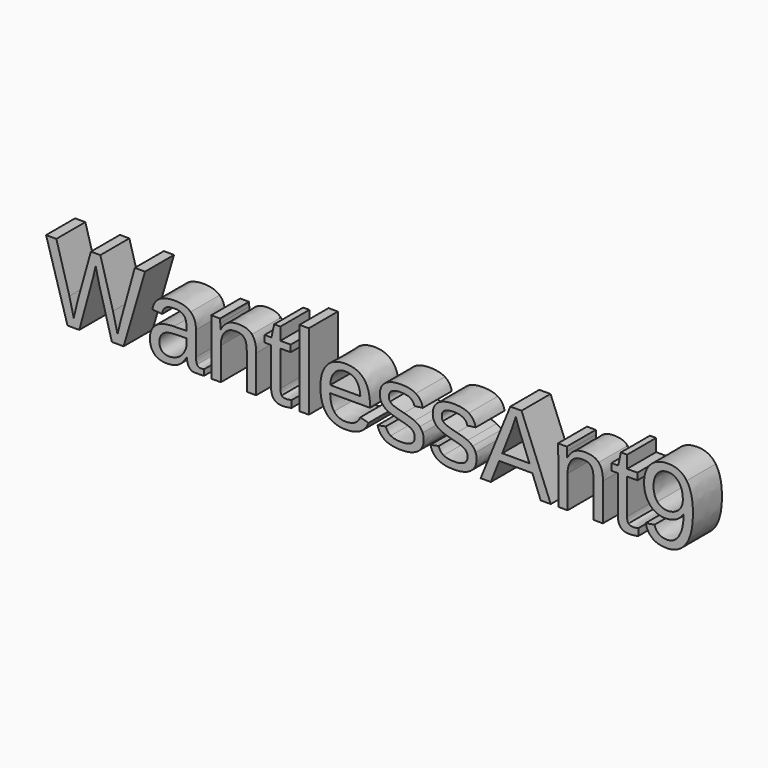
from build123d import *

# Parameters (mm, degrees)
F0_W     = 2.5657552083
F0_H     = 21
F1_DEPTH = 10


with BuildPart() as f1:
    # F0 (on Front) → F1 (new body)
    with BuildSketch(Plane.XZ):
        with BuildLine():
            Line((79.0343266088, 10), (83.371302383, 10))
            add(Edge.make_bspline(
                [(86.66796875, 12.4905598958), (85.3878334896, 10.605916318), (83.371302383, 10)],
                knots=[0, 0, 0, 0.6784981919, 0.6784981919, 0.6784981919], degree=2))
            add(Edge.make_bspline(
                [(88.5546875, 20.4407552083), (88.5546875, 15.2682291667), (86.66796875, 12.4905598958)],
                knots=[0, 0, 0, 1, 1, 1], degree=2))
            add(Edge.make_bspline(
                [(86.83203125, 27.8873697917), (88.5546875, 25.408203125), (88.5546875, 20.4407552083)],
                knots=[0, 0, 0, 1, 1, 1], degree=2))
            add(Edge.make_bspline(
                [(81.7643229167, 30.3665364583), (85.109375, 30.3665364583), (86.83203125, 27.8873697917)],
                knots=[0, 0, 0, 1, 1, 1], degree=2))
            add(Edge.make_bspline(
                [(76.8492838542, 28.5641276042), (78.615234375, 30.3665364583), (81.7643229167, 30.3665364583)],
                knots=[0, 0, 0, 1, 1, 1], degree=2))
            add(Edge.make_bspline(
                [(75.0833333333, 23.6171875), (75.0833333333, 26.76171875), (76.8492838542, 28.5641276042)],
                knots=[0, 0, 0, 1, 1, 1], degree=2))
            add(Edge.make_bspline(
                [(76.7080078125, 18.7021484375), (75.0833333333, 20.5546875), (75.0833333333, 23.6171875)],
                knots=[0, 0, 0, 1, 1, 1], degree=2))
            add(Edge.make_bspline(
                [(81.03515625, 16.849609375), (78.3326822917, 16.849609375), (76.7080078125, 18.7021484375)],
                knots=[0, 0, 0, 1, 1, 1], degree=2))
            add(Edge.make_bspline(
                [(84.0703125, 17.6266276042), (82.689453125, 16.849609375), (81.03515625, 16.849609375)],
                knots=[0, 0, 0, 1, 1, 1], degree=2))
            add(Edge.make_bspline(
                [(86.0208333333, 19.6842447917), (85.451171875, 18.4036458333), (84.0703125, 17.6266276042)],
                knots=[0, 0, 0, 1, 1, 1], degree=2))
            add(Edge.make_bspline(
                [(84.75390625, 13.8326822917), (85.9661458333, 15.8834635417), (86.0208333333, 19.6842447917)],
                knots=[0, 0, 0, 1, 1, 1], degree=2))
            add(Edge.make_bspline(
                [(81.3359375, 11.7819010417), (83.5416666667, 11.7819010417), (84.75390625, 13.8326822917)],
                knots=[0, 0, 0, 1, 1, 1], degree=2))
            add(Edge.make_bspline(
                [(77.9453125, 14.2884114583), (78.7154947917, 11.7819010417), (81.3359375, 11.7819010417)],
                knots=[0, 0, 0, 1, 1, 1], degree=2))
            Line((77.9453125, 14.2884114583), (75.498046875, 13.9010416667))
            add(Edge.make_bspline(
                [(77.5260416667, 10.7041015625), (76.1087239583, 11.6953125), (75.498046875, 13.9010416667)],
                knots=[0, 0, 0, 1, 1, 1], degree=2))
            add(Edge.make_bspline(
                [(79.0343266088, 10), (78.1805643403, 10.2463566059), (77.5260416667, 10.7041015625)],
                knots=[0.5381962211, 0.5381962211, 0.5381962211, 1, 1, 1], degree=2))
        make_face()
        with BuildLine():
            add(Edge.make_bspline(
                [(85.765625, 22.9153645833), (85.765625, 25.33984375), (84.6536458333, 26.8141276042)],
                knots=[0, 0, 0, 1, 1, 1], degree=2))
            add(Edge.make_bspline(
                [(85.2164713542, 20.8098958333), (85.765625, 21.7350260417), (85.765625, 22.9153645833)],
                knots=[0, 0, 0, 1, 1, 1], degree=2))
            add(Edge.make_bspline(
                [(83.7125651042, 19.37890625), (84.6673177083, 19.884765625), (85.2164713542, 20.8098958333)],
                knots=[0, 0, 0, 1, 1, 1], degree=2))
            add(Edge.make_bspline(
                [(81.650390625, 18.873046875), (82.7578125, 18.873046875), (83.7125651042, 19.37890625)],
                knots=[0, 0, 0, 1, 1, 1], degree=2))
            add(Edge.make_bspline(
                [(78.7587890625, 20.1468098958), (79.8274739583, 18.873046875), (81.650390625, 18.873046875)],
                knots=[0, 0, 0, 1, 1, 1], degree=2))
            add(Edge.make_bspline(
                [(77.6901041667, 23.6171875), (77.6901041667, 21.4205729167), (78.7587890625, 20.1468098958)],
                knots=[0, 0, 0, 1, 1, 1], degree=2))
            add(Edge.make_bspline(
                [(78.7587890625, 27.0260416667), (77.6901041667, 25.763671875), (77.6901041667, 23.6171875)],
                knots=[0, 0, 0, 1, 1, 1], degree=2))
            add(Edge.make_bspline(
                [(81.677734375, 28.2884114583), (79.8274739583, 28.2884114583), (78.7587890625, 27.0260416667)],
                knots=[0, 0, 0, 1, 1, 1], degree=2))
            add(Edge.make_bspline(
                [(84.6536458333, 26.8141276042), (83.5416666667, 28.2884114583), (81.677734375, 28.2884114583)],
                knots=[0, 0, 0, 1, 1, 1], degree=2))
        make_face(mode=Mode.SUBTRACT)
        with BuildLine():
            add(Edge.make_bspline(
                [(83.371302383, 10), (82.4157826709, 9.712890625), (81.294921875, 9.712890625)],
                knots=[0.6784981919, 0.6784981919, 0.6784981919, 1, 1, 1], degree=2))
            Line((83.371302383, 10), (79.0343266088, 10))
            add(Edge.make_bspline(
                [(81.294921875, 9.712890625), (80.0293198238, 9.712890625), (79.0343266088, 10)],
                knots=[0, 0, 0, 0.5381962211, 0.5381962211, 0.5381962211], degree=2))
        make_face()
        with BuildLine():
            add(Edge.make_bspline(
                [(73.0351407022, 10), (71.9925052469, 9.7721354167), (70.9134114583, 9.7721354167)],
                knots=[0.1835034191, 0.1835034191, 0.1835034191, 1, 1, 1], degree=2))
            Line((73.0351407022, 10), (69.5423555663, 10))
            add(Edge.make_bspline(
                [(70.9134114583, 9.7721354167), (70.1274862579, 9.7721354167), (69.5423555663, 10)],
                knots=[0, 0, 0, 0.2554880652, 0.2554880652, 0.2554880652], degree=2))
        make_face()
        with BuildLine():
            Line((69.5423555663, 10), (73.0351407022, 10))
            add(Edge.make_bspline(
                [(73.501953125, 10.1139322917), (73.2694676735, 10.0512113965), (73.0351407022, 10)],
                knots=[0, 0, 0, 0.1835034191, 0.1835034191, 0.1835034191], degree=2))
            Line((73.501953125, 10.1139322917), (73.501953125, 12.009765625))
            add(Edge.make_bspline(
                [(72.0208333333, 11.8092447917), (72.5358072917, 11.8092447917), (73.501953125, 12.009765625)],
                knots=[0, 0, 0, 1, 1, 1], degree=2))
            add(Edge.make_bspline(
                [(70.7607421875, 12.2581380208), (71.123046875, 11.8092447917), (72.0208333333, 11.8092447917)],
                knots=[0, 0, 0, 1, 1, 1], degree=2))
            add(Edge.make_bspline(
                [(70.3984375, 13.8190104167), (70.3984375, 12.70703125), (70.7607421875, 12.2581380208)],
                knots=[0, 0, 0, 1, 1, 1], degree=2))
            Line((70.3984375, 13.8190104167), (70.3984375, 23.5442708333))
            Line((70.3984375, 23.5442708333), (73.2467447917, 23.5442708333))
            Line((73.2467447917, 23.5442708333), (73.2467447917, 25.408203125))
            Line((73.2467447917, 25.408203125), (70.3984375, 25.408203125))
            Line((70.3984375, 25.408203125), (70.3984375, 28.8580729167))
            Line((70.3984375, 28.8580729167), (68.689453125, 28.8580729167))
            Line((68.689453125, 28.8580729167), (67.9329427083, 25.408203125))
            Line((67.9329427083, 25.408203125), (66.0553385417, 25.408203125))
            Line((66.0553385417, 25.408203125), (66.0553385417, 23.5442708333))
            Line((66.0553385417, 23.5442708333), (67.8372395833, 23.5442708333))
            Line((67.8372395833, 23.5442708333), (67.8372395833, 13.2630208333))
            add(Edge.make_bspline(
                [(69.5423555663, 10), (67.8372395833, 10.6640149774), (67.8372395833, 13.2630208333)],
                knots=[0.2554880652, 0.2554880652, 0.2554880652, 1, 1, 1], degree=2))
        make_face()
        with BuildLine():
            Line((61.142578125, 10), (63.7220052083, 10))
            Line((63.7220052083, 10), (63.7220052083, 20.267578125))
            add(Edge.make_bspline(
                [(62.5462239583, 24.4352213542), (63.7220052083, 23.1751302083), (63.7220052083, 20.267578125)],
                knots=[0, 0, 0, 1, 1, 1], degree=2))
            add(Edge.make_bspline(
                [(58.8365885417, 25.6953125), (61.3704427083, 25.6953125), (62.5462239583, 24.4352213542)],
                knots=[0, 0, 0, 1, 1, 1], degree=2))
            add(Edge.make_bspline(
                [(55.9518229167, 25.0322265625), (57.1139322917, 25.6953125), (58.8365885417, 25.6953125)],
                knots=[0, 0, 0, 1, 1, 1], degree=2))
            add(Edge.make_bspline(
                [(53.91015625, 22.7740885417), (54.7897135417, 24.369140625), (55.9518229167, 25.0322265625)],
                knots=[0, 0, 0, 1, 1, 1], degree=2))
            Line((53.91015625, 22.7740885417), (53.8645833333, 22.7740885417))
            add(Edge.make_bspline(
                [(53.8167317708, 24.3053385417), (53.8372395833, 23.8997395833), (53.8645833333, 22.7740885417)],
                knots=[0, 0, 0, 1, 1, 1], degree=2))
            add(Edge.make_bspline(
                [(53.7802734375, 25.025390625), (53.7962239583, 24.7109375), (53.8167317708, 24.3053385417)],
                knots=[0, 0, 0, 1, 1, 1], degree=2))
            add(Edge.make_bspline(
                [(53.7506510417, 25.408203125), (53.7643229167, 25.33984375), (53.7802734375, 25.025390625)],
                knots=[0, 0, 0, 1, 1, 1], degree=2))
            Line((53.7506510417, 25.408203125), (51.3307291667, 25.408203125))
            add(Edge.make_bspline(
                [(51.4173177083, 22.1178385417), (51.4173177083, 24.8111979167), (51.3307291667, 25.408203125)],
                knots=[0, 0, 0, 1, 1, 1], degree=2))
            Line((51.4173177083, 22.1178385417), (51.4173177083, 10))
            Line((51.4173177083, 10), (53.978515625, 10))
            Line((53.978515625, 10), (53.978515625, 18.927734375))
            add(Edge.make_bspline(
                [(55.0472005208, 22.4459635417), (53.978515625, 21.1790364583), (53.978515625, 18.927734375)],
                knots=[0, 0, 0, 1, 1, 1], degree=2))
            add(Edge.make_bspline(
                [(57.9661458333, 23.712890625), (56.1158854167, 23.712890625), (55.0472005208, 22.4459635417)],
                knots=[0, 0, 0, 1, 1, 1], degree=2))
            add(Edge.make_bspline(
                [(59.8893229167, 23.34375), (59.2330729167, 23.712890625), (57.9661458333, 23.712890625)],
                knots=[0, 0, 0, 1, 1, 1], degree=2))
            add(Edge.make_bspline(
                [(60.8440755208, 22.1337890625), (60.5455729167, 22.974609375), (59.8893229167, 23.34375)],
                knots=[0, 0, 0, 1, 1, 1], degree=2))
            add(Edge.make_bspline(
                [(61.142578125, 19.7708333333), (61.142578125, 21.29296875), (60.8440755208, 22.1337890625)],
                knots=[0, 0, 0, 1, 1, 1], degree=2))
            Line((61.142578125, 19.7708333333), (61.142578125, 10))
        make_face()
        Polygon((38.1829427083, 30.0657552083), (29.998046875, 10), (32.814453125, 10), (35.125, 15.8697916667), (44.2669270833, 15.8697916667), (46.5592447917, 10), (49.3346354167, 10), (41.27734375, 30.0657552083), align=None)
        with BuildLine():
            Line((39.568359375, 27.6184895833), (39.6959635417, 28.0149739583))
            Line((39.6959635417, 28.0149739583), (40.0787760417, 26.8346354167))
            add(Edge.make_bspline(
                [(40.8763020833, 24.6106770833), (40.4798177083, 25.5950520833), (40.0787760417, 26.8346354167)],
                knots=[0, 0, 0, 1, 1, 1], degree=2))
            Line((40.8763020833, 24.6106770833), (43.4557291667, 17.9889322917))
            Line((43.4557291667, 17.9889322917), (35.9498697917, 17.9889322917))
            Line((35.9498697917, 17.9889322917), (38.5110677083, 24.5833333333))
            add(Edge.make_bspline(
                [(39.568359375, 27.6184895833), (39.2083333333, 26.43359375), (38.5110677083, 24.5833333333)],
                knots=[0, 0, 0, 1, 1, 1], degree=2))
        make_face(mode=Mode.SUBTRACT)
        with BuildLine():
            add(Edge.make_bspline(
                [(19.8664633143, 10), (18.8987870961, 10.2345761258), (18.1969401042, 10.6608072917)],
                knots=[0.5503495393, 0.5503495393, 0.5503495393, 1, 1, 1], degree=2))
            Line((19.8664633143, 10), (25.2328343309, 10))
            add(Edge.make_bspline(
                [(27.2408854167, 10.8955078125), (26.4063199616, 10.2955916475), (25.2328343309, 10)],
                knots=[0, 0, 0, 0.5072784088, 0.5072784088, 0.5072784088], degree=2))
            add(Edge.make_bspline(
                [(28.8860677083, 14.2565104167), (28.8860677083, 12.078125), (27.2408854167, 10.8955078125)],
                knots=[0, 0, 0, 1, 1, 1], degree=2))
            add(Edge.make_bspline(
                [(28.6012369792, 15.8310546875), (28.8860677083, 15.140625), (28.8860677083, 14.2565104167)],
                knots=[0, 0, 0, 1, 1, 1], degree=2))
            add(Edge.make_bspline(
                [(27.796875, 17.0501302083), (28.31640625, 16.521484375), (28.6012369792, 15.8310546875)],
                knots=[0, 0, 0, 1, 1, 1], degree=2))
            add(Edge.make_bspline(
                [(26.3795572917, 18.01171875), (27.27734375, 17.5787760417), (27.796875, 17.0501302083)],
                knots=[0, 0, 0, 1, 1, 1], degree=2))
            add(Edge.make_bspline(
                [(23.4446614583, 18.9596354167), (25.4817708333, 18.4446614583), (26.3795572917, 18.01171875)],
                knots=[0, 0, 0, 1, 1, 1], degree=2))
            add(Edge.make_bspline(
                [(20.6236979167, 19.7845052083), (21.2936197917, 19.4837239583), (23.4446614583, 18.9596354167)],
                knots=[0, 0, 0, 1, 1, 1], degree=2))
            add(Edge.make_bspline(
                [(19.6119791667, 20.5113932292), (19.9537760417, 20.0852864583), (20.6236979167, 19.7845052083)],
                knots=[0, 0, 0, 1, 1, 1], degree=2))
            add(Edge.make_bspline(
                [(19.2701822917, 21.59375), (19.2701822917, 20.9375), (19.6119791667, 20.5113932292)],
                knots=[0, 0, 0, 1, 1, 1], degree=2))
            add(Edge.make_bspline(
                [(20.0973307292, 23.1865234375), (19.2701822917, 22.66015625), (19.2701822917, 21.59375)],
                knots=[0, 0, 0, 1, 1, 1], degree=2))
            add(Edge.make_bspline(
                [(22.6608072917, 23.712890625), (20.9244791667, 23.712890625), (20.0973307292, 23.1865234375)],
                knots=[0, 0, 0, 1, 1, 1], degree=2))
            add(Edge.make_bspline(
                [(25.1604817708, 23.166015625), (24.228515625, 23.712890625), (22.6608072917, 23.712890625)],
                knots=[0, 0, 0, 1, 1, 1], degree=2))
            add(Edge.make_bspline(
                [(26.306640625, 21.59375), (26.0924479167, 22.619140625), (25.1604817708, 23.166015625)],
                knots=[0, 0, 0, 1, 1, 1], degree=2))
            Line((26.306640625, 21.59375), (28.6126302083, 21.8763020833))
            add(Edge.make_bspline(
                [(26.7145182292, 24.7542317708), (28.2161458333, 23.8587239583), (28.6126302083, 21.8763020833)],
                knots=[0, 0, 0, 1, 1, 1], degree=2))
            add(Edge.make_bspline(
                [(22.6608072917, 25.6497395833), (25.212890625, 25.6497395833), (26.7145182292, 24.7542317708)],
                knots=[0, 0, 0, 1, 1, 1], degree=2))
            add(Edge.make_bspline(
                [(18.2835286458, 24.546875), (19.78515625, 25.6497395833), (22.6608072917, 25.6497395833)],
                knots=[0, 0, 0, 1, 1, 1], degree=2))
            add(Edge.make_bspline(
                [(16.7819010417, 21.3385416667), (16.7819010417, 23.4440104167), (18.2835286458, 24.546875)],
                knots=[0, 0, 0, 1, 1, 1], degree=2))
            add(Edge.make_bspline(
                [(17.3082682292, 19.4153645833), (16.7819010417, 20.19921875), (16.7819010417, 21.3385416667)],
                knots=[0, 0, 0, 1, 1, 1], degree=2))
            add(Edge.make_bspline(
                [(18.7666015625, 18.0823567708), (17.8346354167, 18.6315104167), (17.3082682292, 19.4153645833)],
                knots=[0, 0, 0, 1, 1, 1], degree=2))
            add(Edge.make_bspline(
                [(21.9088541667, 16.9635416667), (19.6985677083, 17.533203125), (18.7666015625, 18.0823567708)],
                knots=[0, 0, 0, 1, 1, 1], degree=2))
            Line((21.9088541667, 16.9635416667), (23.7454427083, 16.48046875))
            add(Edge.make_bspline(
                [(25.7666015625, 15.5416666667), (25.1399739583, 16.111328125), (23.7454427083, 16.48046875)],
                knots=[0, 0, 0, 1, 1, 1], degree=2))
            add(Edge.make_bspline(
                [(26.3932291667, 14.060546875), (26.3932291667, 14.9720052083), (25.7666015625, 15.5416666667)],
                knots=[0, 0, 0, 1, 1, 1], degree=2))
            add(Edge.make_bspline(
                [(25.4886067708, 12.2649739583), (26.3932291667, 12.8619791667), (26.3932291667, 14.060546875)],
                knots=[0, 0, 0, 1, 1, 1], degree=2))
            add(Edge.make_bspline(
                [(22.6334635417, 11.66796875), (24.583984375, 11.66796875), (25.4886067708, 12.2649739583)],
                knots=[0, 0, 0, 1, 1, 1], degree=2))
            add(Edge.make_bspline(
                [(19.78515625, 12.2444661458), (20.810546875, 11.66796875), (22.6334635417, 11.66796875)],
                knots=[0, 0, 0, 1, 1, 1], degree=2))
            add(Edge.make_bspline(
                [(18.431640625, 14.060546875), (18.759765625, 12.8209635417), (19.78515625, 12.2444661458)],
                knots=[0, 0, 0, 1, 1, 1], degree=2))
            Line((18.431640625, 14.060546875), (16.1666666667, 13.6184895833))
            add(Edge.make_bspline(
                [(18.1969401042, 10.6608072917), (16.6360677083, 11.6087239583), (16.1666666667, 13.6184895833)],
                knots=[0, 0, 0, 1, 1, 1], degree=2))
        make_face()
        with BuildLine():
            add(Edge.make_bspline(
                [(5.283129981, 10), (4.3154537627, 10.2345761258), (3.6136067708, 10.6608072917)],
                knots=[0.5503495393, 0.5503495393, 0.5503495393, 1, 1, 1], degree=2))
            Line((5.283129981, 10), (10.6495009976, 10))
            add(Edge.make_bspline(
                [(12.6575520833, 10.8955078125), (11.8229866283, 10.2955916475), (10.6495009976, 10)],
                knots=[0, 0, 0, 0.5072784088, 0.5072784088, 0.5072784088], degree=2))
            add(Edge.make_bspline(
                [(14.302734375, 14.2565104167), (14.302734375, 12.078125), (12.6575520833, 10.8955078125)],
                knots=[0, 0, 0, 1, 1, 1], degree=2))
            add(Edge.make_bspline(
                [(14.0179036458, 15.8310546875), (14.302734375, 15.140625), (14.302734375, 14.2565104167)],
                knots=[0, 0, 0, 1, 1, 1], degree=2))
            add(Edge.make_bspline(
                [(13.2135416667, 17.0501302083), (13.7330729167, 16.521484375), (14.0179036458, 15.8310546875)],
                knots=[0, 0, 0, 1, 1, 1], degree=2))
            add(Edge.make_bspline(
                [(11.7962239583, 18.01171875), (12.6940104167, 17.5787760417), (13.2135416667, 17.0501302083)],
                knots=[0, 0, 0, 1, 1, 1], degree=2))
            add(Edge.make_bspline(
                [(8.861328125, 18.9596354167), (10.8984375, 18.4446614583), (11.7962239583, 18.01171875)],
                knots=[0, 0, 0, 1, 1, 1], degree=2))
            add(Edge.make_bspline(
                [(6.0403645833, 19.7845052083), (6.7102864583, 19.4837239583), (8.861328125, 18.9596354167)],
                knots=[0, 0, 0, 1, 1, 1], degree=2))
            add(Edge.make_bspline(
                [(5.0286458333, 20.5113932292), (5.3704427083, 20.0852864583), (6.0403645833, 19.7845052083)],
                knots=[0, 0, 0, 1, 1, 1], degree=2))
            add(Edge.make_bspline(
                [(4.6868489583, 21.59375), (4.6868489583, 20.9375), (5.0286458333, 20.5113932292)],
                knots=[0, 0, 0, 1, 1, 1], degree=2))
            add(Edge.make_bspline(
                [(5.5139973958, 23.1865234375), (4.6868489583, 22.66015625), (4.6868489583, 21.59375)],
                knots=[0, 0, 0, 1, 1, 1], degree=2))
            add(Edge.make_bspline(
                [(8.0774739583, 23.712890625), (6.3411458333, 23.712890625), (5.5139973958, 23.1865234375)],
                knots=[0, 0, 0, 1, 1, 1], degree=2))
            add(Edge.make_bspline(
                [(10.5771484375, 23.166015625), (9.6451822917, 23.712890625), (8.0774739583, 23.712890625)],
                knots=[0, 0, 0, 1, 1, 1], degree=2))
            add(Edge.make_bspline(
                [(11.7233072917, 21.59375), (11.5091145833, 22.619140625), (10.5771484375, 23.166015625)],
                knots=[0, 0, 0, 1, 1, 1], degree=2))
            Line((11.7233072917, 21.59375), (14.029296875, 21.8763020833))
            add(Edge.make_bspline(
                [(12.1311848958, 24.7542317708), (13.6328125, 23.8587239583), (14.029296875, 21.8763020833)],
                knots=[0, 0, 0, 1, 1, 1], degree=2))
            add(Edge.make_bspline(
                [(8.0774739583, 25.6497395833), (10.6295572917, 25.6497395833), (12.1311848958, 24.7542317708)],
                knots=[0, 0, 0, 1, 1, 1], degree=2))
            add(Edge.make_bspline(
                [(3.7001953125, 24.546875), (5.2018229167, 25.6497395833), (8.0774739583, 25.6497395833)],
                knots=[0, 0, 0, 1, 1, 1], degree=2))
            add(Edge.make_bspline(
                [(2.1985677083, 21.3385416667), (2.1985677083, 23.4440104167), (3.7001953125, 24.546875)],
                knots=[0, 0, 0, 1, 1, 1], degree=2))
            add(Edge.make_bspline(
                [(2.7249348958, 19.4153645833), (2.1985677083, 20.19921875), (2.1985677083, 21.3385416667)],
                knots=[0, 0, 0, 1, 1, 1], degree=2))
            add(Edge.make_bspline(
                [(4.1832682292, 18.0823567708), (3.2513020833, 18.6315104167), (2.7249348958, 19.4153645833)],
                knots=[0, 0, 0, 1, 1, 1], degree=2))
            add(Edge.make_bspline(
                [(7.3255208333, 16.9635416667), (5.115234375, 17.533203125), (4.1832682292, 18.0823567708)],
                knots=[0, 0, 0, 1, 1, 1], degree=2))
            Line((7.3255208333, 16.9635416667), (9.162109375, 16.48046875))
            add(Edge.make_bspline(
                [(11.1832682292, 15.5416666667), (10.556640625, 16.111328125), (9.162109375, 16.48046875)],
                knots=[0, 0, 0, 1, 1, 1], degree=2))
            add(Edge.make_bspline(
                [(11.8098958333, 14.060546875), (11.8098958333, 14.9720052083), (11.1832682292, 15.5416666667)],
                knots=[0, 0, 0, 1, 1, 1], degree=2))
            add(Edge.make_bspline(
                [(10.9052734375, 12.2649739583), (11.8098958333, 12.8619791667), (11.8098958333, 14.060546875)],
                knots=[0, 0, 0, 1, 1, 1], degree=2))
            add(Edge.make_bspline(
                [(8.0501302083, 11.66796875), (10.0006510417, 11.66796875), (10.9052734375, 12.2649739583)],
                knots=[0, 0, 0, 1, 1, 1], degree=2))
            add(Edge.make_bspline(
                [(5.2018229167, 12.2444661458), (6.2272135417, 11.66796875), (8.0501302083, 11.66796875)],
                knots=[0, 0, 0, 1, 1, 1], degree=2))
            add(Edge.make_bspline(
                [(3.8483072917, 14.060546875), (4.1764322917, 12.8209635417), (5.2018229167, 12.2444661458)],
                knots=[0, 0, 0, 1, 1, 1], degree=2))
            Line((3.8483072917, 14.060546875), (1.5833333333, 13.6184895833))
            add(Edge.make_bspline(
                [(3.6136067708, 10.6608072917), (2.052734375, 11.6087239583), (1.5833333333, 13.6184895833)],
                knots=[0, 0, 0, 1, 1, 1], degree=2))
        make_face()
        with BuildLine():
            Line((25.2328343309, 10), (19.8664633143, 10))
            add(Edge.make_bspline(
                [(22.6334635417, 9.712890625), (21.0508503158, 9.712890625), (19.8664633143, 10)],
                knots=[0, 0, 0, 0.5503495393, 0.5503495393, 0.5503495393], degree=2))
            add(Edge.make_bspline(
                [(25.2328343309, 10), (24.0930229428, 9.712890625), (22.6334635417, 9.712890625)],
                knots=[0.5072784088, 0.5072784088, 0.5072784088, 1, 1, 1], degree=2))
        make_face()
        with BuildLine():
            Line((10.6495009976, 10), (5.283129981, 10))
            add(Edge.make_bspline(
                [(8.0501302083, 9.712890625), (6.4675169824, 9.712890625), (5.283129981, 10)],
                knots=[0, 0, 0, 0.5503495393, 0.5503495393, 0.5503495393], degree=2))
            add(Edge.make_bspline(
                [(10.6495009976, 10), (9.5096896095, 9.712890625), (8.0501302083, 9.712890625)],
                knots=[0.5072784088, 0.5072784088, 0.5072784088, 1, 1, 1], degree=2))
        make_face()
        with BuildLine():
            Line((-4.7456217987, 10), (-9.5531948379, 10))
            add(Edge.make_bspline(
                [(-7.216796875, 9.712890625), (-8.499968067, 9.712890625), (-9.5531948379, 10)],
                knots=[0, 0, 0, 0.3754192288, 0.3754192288, 0.3754192288], degree=2))
            add(Edge.make_bspline(
                [(-4.7456217987, 10), (-5.8428520101, 9.712890625), (-7.216796875, 9.712890625)],
                knots=[0.7195509219, 0.7195509219, 0.7195509219, 1, 1, 1], degree=2))
        make_face()
        with BuildLine():
            add(Edge.make_bspline(
                [(-9.5531948379, 10), (-11.3054364347, 10.4776606554), (-12.4212239583, 11.75)],
                knots=[0.3754192288, 0.3754192288, 0.3754192288, 1, 1, 1], degree=2))
            Line((-9.5531948379, 10), (-4.7456217987, 10))
            add(Edge.make_bspline(
                [(-0.9368489583, 13.36328125), (-1.9304475947, 10.7366393104), (-4.7456217987, 10)],
                knots=[0, 0, 0, 0.7195509219, 0.7195509219, 0.7195509219], degree=2))
            Line((-0.9368489583, 13.36328125), (-3.18359375, 14.0013020833))
            add(Edge.make_bspline(
                [(-4.5439453125, 12.3059895833), (-3.5390625, 12.9759114583), (-3.18359375, 14.0013020833)],
                knots=[0, 0, 0, 1, 1, 1], degree=2))
            add(Edge.make_bspline(
                [(-7.216796875, 11.6360677083), (-5.548828125, 11.6360677083), (-4.5439453125, 12.3059895833)],
                knots=[0, 0, 0, 1, 1, 1], degree=2))
            add(Edge.make_bspline(
                [(-10.4182942708, 13.076171875), (-9.322265625, 11.6360677083), (-7.216796875, 11.6360677083)],
                knots=[0, 0, 0, 1, 1, 1], degree=2))
            add(Edge.make_bspline(
                [(-11.5143229167, 17.1640625), (-11.5143229167, 14.5162760417), (-10.4182942708, 13.076171875)],
                knots=[0, 0, 0, 1, 1, 1], degree=2))
            Line((-11.5143229167, 17.1640625), (-0.5221354167, 17.1640625))
            Line((-0.5221354167, 17.1640625), (-0.5221354167, 17.505859375))
            add(Edge.make_bspline(
                [(-7.3170572917, 25.6953125), (-0.5221354167, 25.6953125), (-0.5221354167, 17.505859375)],
                knots=[0, 0, 0, 1, 1, 1], degree=2))
            add(Edge.make_bspline(
                [(-12.4212239583, 23.658203125), (-10.634765625, 25.6953125), (-7.3170572917, 25.6953125)],
                knots=[0, 0, 0, 1, 1, 1], degree=2))
            add(Edge.make_bspline(
                [(-14.2076822917, 17.806640625), (-14.2076822917, 21.62109375), (-12.4212239583, 23.658203125)],
                knots=[0, 0, 0, 1, 1, 1], degree=2))
            add(Edge.make_bspline(
                [(-12.4212239583, 11.75), (-14.2076822917, 13.787109375), (-14.2076822917, 17.806640625)],
                knots=[0, 0, 0, 1, 1, 1], degree=2))
        make_face()
        with BuildLine():
            add(Edge.make_bspline(
                [(-3.169921875, 19.1282552083), (-3.3841145833, 21.56640625), (-4.4095052083, 22.6829427083)],
                knots=[0, 0, 0, 1, 1, 1], degree=2))
            Line((-3.169921875, 19.1282552083), (-11.4869791667, 19.1282552083))
            add(Edge.make_bspline(
                [(-10.3111979167, 22.5530598958), (-11.400390625, 21.306640625), (-11.4869791667, 19.1282552083)],
                knots=[0, 0, 0, 1, 1, 1], degree=2))
            add(Edge.make_bspline(
                [(-7.3580729167, 23.7994791667), (-9.2220052083, 23.7994791667), (-10.3111979167, 22.5530598958)],
                knots=[0, 0, 0, 1, 1, 1], degree=2))
            add(Edge.make_bspline(
                [(-4.4095052083, 22.6829427083), (-5.4348958333, 23.7994791667), (-7.3580729167, 23.7994791667)],
                knots=[0, 0, 0, 1, 1, 1], degree=2))
        make_face(mode=Mode.SUBTRACT)
        with Locations((-18.6806640625, 20.5)):
            Rectangle(F0_W, F0_H)
        with BuildLine():
            Line((-26.101524642, 10), (-22.6087395061, 10))
            add(Edge.make_bspline(
                [(-22.1419270833, 10.1139322917), (-22.3744125348, 10.0512113965), (-22.6087395061, 10)],
                knots=[0, 0, 0, 0.1835034191, 0.1835034191, 0.1835034191], degree=2))
            Line((-22.1419270833, 10.1139322917), (-22.1419270833, 12.009765625))
            add(Edge.make_bspline(
                [(-23.623046875, 11.8092447917), (-23.1080729167, 11.8092447917), (-22.1419270833, 12.009765625)],
                knots=[0, 0, 0, 1, 1, 1], degree=2))
            add(Edge.make_bspline(
                [(-24.8831380208, 12.2581380208), (-24.5208333333, 11.8092447917), (-23.623046875, 11.8092447917)],
                knots=[0, 0, 0, 1, 1, 1], degree=2))
            add(Edge.make_bspline(
                [(-25.2454427083, 13.8190104167), (-25.2454427083, 12.70703125), (-24.8831380208, 12.2581380208)],
                knots=[0, 0, 0, 1, 1, 1], degree=2))
            Line((-25.2454427083, 13.8190104167), (-25.2454427083, 23.5442708333))
            Line((-25.2454427083, 23.5442708333), (-22.3971354167, 23.5442708333))
            Line((-22.3971354167, 23.5442708333), (-22.3971354167, 25.408203125))
            Line((-22.3971354167, 25.408203125), (-25.2454427083, 25.408203125))
            Line((-25.2454427083, 25.408203125), (-25.2454427083, 28.8580729167))
            Line((-25.2454427083, 28.8580729167), (-26.9544270833, 28.8580729167))
            Line((-26.9544270833, 28.8580729167), (-27.7109375, 25.408203125))
            Line((-27.7109375, 25.408203125), (-29.5885416667, 25.408203125))
            Line((-29.5885416667, 25.408203125), (-29.5885416667, 23.5442708333))
            Line((-29.5885416667, 23.5442708333), (-27.806640625, 23.5442708333))
            Line((-27.806640625, 23.5442708333), (-27.806640625, 13.2630208333))
            add(Edge.make_bspline(
                [(-26.101524642, 10), (-27.806640625, 10.6640149774), (-27.806640625, 13.2630208333)],
                knots=[0.2554880652, 0.2554880652, 0.2554880652, 1, 1, 1], degree=2))
        make_face()
        with BuildLine():
            add(Edge.make_bspline(
                [(-22.6087395061, 10), (-23.6513749614, 9.7721354167), (-24.73046875, 9.7721354167)],
                knots=[0.1835034191, 0.1835034191, 0.1835034191, 1, 1, 1], degree=2))
            Line((-22.6087395061, 10), (-26.101524642, 10))
            add(Edge.make_bspline(
                [(-24.73046875, 9.7721354167), (-25.5163939504, 9.7721354167), (-26.101524642, 10)],
                knots=[0, 0, 0, 0.2554880652, 0.2554880652, 0.2554880652], degree=2))
        make_face()
        with BuildLine():
            Line((-34.5013020833, 10), (-31.921875, 10))
            Line((-31.921875, 10), (-31.921875, 20.267578125))
            add(Edge.make_bspline(
                [(-33.09765625, 24.4352213542), (-31.921875, 23.1751302083), (-31.921875, 20.267578125)],
                knots=[0, 0, 0, 1, 1, 1], degree=2))
            add(Edge.make_bspline(
                [(-36.8072916667, 25.6953125), (-34.2734375, 25.6953125), (-33.09765625, 24.4352213542)],
                knots=[0, 0, 0, 1, 1, 1], degree=2))
            add(Edge.make_bspline(
                [(-39.6920572917, 25.0322265625), (-38.5299479167, 25.6953125), (-36.8072916667, 25.6953125)],
                knots=[0, 0, 0, 1, 1, 1], degree=2))
            add(Edge.make_bspline(
                [(-41.7337239583, 22.7740885417), (-40.8541666667, 24.369140625), (-39.6920572917, 25.0322265625)],
                knots=[0, 0, 0, 1, 1, 1], degree=2))
            Line((-41.7337239583, 22.7740885417), (-41.779296875, 22.7740885417))
            add(Edge.make_bspline(
                [(-41.8271484375, 24.3053385417), (-41.806640625, 23.8997395833), (-41.779296875, 22.7740885417)],
                knots=[0, 0, 0, 1, 1, 1], degree=2))
            add(Edge.make_bspline(
                [(-41.8636067708, 25.025390625), (-41.84765625, 24.7109375), (-41.8271484375, 24.3053385417)],
                knots=[0, 0, 0, 1, 1, 1], degree=2))
            add(Edge.make_bspline(
                [(-41.8932291667, 25.408203125), (-41.8795572917, 25.33984375), (-41.8636067708, 25.025390625)],
                knots=[0, 0, 0, 1, 1, 1], degree=2))
            Line((-41.8932291667, 25.408203125), (-44.3131510417, 25.408203125))
            add(Edge.make_bspline(
                [(-44.2265625, 22.1178385417), (-44.2265625, 24.8111979167), (-44.3131510417, 25.408203125)],
                knots=[0, 0, 0, 1, 1, 1], degree=2))
            Line((-44.2265625, 22.1178385417), (-44.2265625, 10))
            Line((-44.2265625, 10), (-41.6653645833, 10))
            Line((-41.6653645833, 10), (-41.6653645833, 18.927734375))
            add(Edge.make_bspline(
                [(-40.5966796875, 22.4459635417), (-41.6653645833, 21.1790364583), (-41.6653645833, 18.927734375)],
                knots=[0, 0, 0, 1, 1, 1], degree=2))
            add(Edge.make_bspline(
                [(-37.677734375, 23.712890625), (-39.5279947917, 23.712890625), (-40.5966796875, 22.4459635417)],
                knots=[0, 0, 0, 1, 1, 1], degree=2))
            add(Edge.make_bspline(
                [(-35.7545572917, 23.34375), (-36.4108072917, 23.712890625), (-37.677734375, 23.712890625)],
                knots=[0, 0, 0, 1, 1, 1], degree=2))
            add(Edge.make_bspline(
                [(-34.7998046875, 22.1337890625), (-35.0983072917, 22.974609375), (-35.7545572917, 23.34375)],
                knots=[0, 0, 0, 1, 1, 1], degree=2))
            add(Edge.make_bspline(
                [(-34.5013020833, 19.7708333333), (-34.5013020833, 21.29296875), (-34.7998046875, 22.1337890625)],
                knots=[0, 0, 0, 1, 1, 1], degree=2))
            Line((-34.5013020833, 19.7708333333), (-34.5013020833, 10))
        make_face()
        with BuildLine():
            Line((-49.318225973, 10), (-46.6628635109, 10))
            add(Edge.make_bspline(
                [(-46.25, 10.0865885417), (-46.4554018434, 10.0381447107), (-46.6628635109, 10)],
                knots=[0, 0, 0, 0.2125992126, 0.2125992126, 0.2125992126], degree=2))
            Line((-46.25, 10.0865885417), (-46.25, 11.681640625))
            add(Edge.make_bspline(
                [(-47.0885416667, 11.5813802083), (-46.7194010417, 11.5813802083), (-46.25, 11.681640625)],
                knots=[0, 0, 0, 1, 1, 1], degree=2))
            add(Edge.make_bspline(
                [(-48.2278645833, 12.1578776042), (-47.9270833333, 11.5813802083), (-47.0885416667, 11.5813802083)],
                knots=[0, 0, 0, 1, 1, 1], degree=2))
            add(Edge.make_bspline(
                [(-48.5286458333, 13.8736979167), (-48.5286458333, 12.734375), (-48.2278645833, 12.1578776042)],
                knots=[0, 0, 0, 1, 1, 1], degree=2))
            Line((-48.5286458333, 13.8736979167), (-48.5286458333, 20.5091145833))
            add(Edge.make_bspline(
                [(-49.9938151042, 24.3623046875), (-48.5286458333, 23.029296875), (-48.5286458333, 20.5091145833)],
                knots=[0, 0, 0, 1, 1, 1], degree=2))
            add(Edge.make_bspline(
                [(-54.3665364583, 25.6953125), (-51.458984375, 25.6953125), (-49.9938151042, 24.3623046875)],
                knots=[0, 0, 0, 1, 1, 1], degree=2))
            add(Edge.make_bspline(
                [(-60.5462239583, 21.5345052083), (-59.8899739583, 25.6953125), (-54.3665364583, 25.6953125)],
                knots=[0, 0, 0, 1, 1, 1], degree=2))
            Line((-60.5462239583, 21.5345052083), (-57.87109375, 21.29296875))
            add(Edge.make_bspline(
                [(-56.927734375, 23.1591796875), (-57.7115885417, 22.5735677083), (-57.87109375, 21.29296875)],
                knots=[0, 0, 0, 1, 1, 1], degree=2))
            add(Edge.make_bspline(
                [(-54.4212239583, 23.7447916667), (-56.1438802083, 23.7447916667), (-56.927734375, 23.1591796875)],
                knots=[0, 0, 0, 1, 1, 1], degree=2))
            add(Edge.make_bspline(
                [(-51.9147135417, 22.9313151042), (-52.7122395833, 23.7447916667), (-54.4212239583, 23.7447916667)],
                knots=[0, 0, 0, 1, 1, 1], degree=2))
            add(Edge.make_bspline(
                [(-51.1171875, 20.240234375), (-51.1171875, 22.1178385417), (-51.9147135417, 22.9313151042)],
                knots=[0, 0, 0, 1, 1, 1], degree=2))
            Line((-51.1171875, 20.240234375), (-51.1171875, 19.4016927083))
            Line((-51.1171875, 19.4016927083), (-54.5807291667, 19.3424479167))
            add(Edge.make_bspline(
                [(-59.6552734375, 17.9752604167), (-58.0807291667, 19.255859375), (-54.5807291667, 19.3424479167)],
                knots=[0, 0, 0, 1, 1, 1], degree=2))
            add(Edge.make_bspline(
                [(-61.2298177083, 14.3020833333), (-61.2298177083, 16.6946614583), (-59.6552734375, 17.9752604167)],
                knots=[0, 0, 0, 1, 1, 1], degree=2))
            add(Edge.make_bspline(
                [(-60.0631510417, 10.9388020833), (-61.2298177083, 12.1647135417), (-61.2298177083, 14.3020833333)],
                knots=[0, 0, 0, 1, 1, 1], degree=2))
            add(Edge.make_bspline(
                [(-58.5507444533, 10), (-59.4610844407, 10.3061617878), (-60.0631510417, 10.9388020833)],
                knots=[0.4839429135, 0.4839429135, 0.4839429135, 1, 1, 1], degree=2))
            Line((-58.5507444533, 10), (-54.4596695565, 10))
            add(Edge.make_bspline(
                [(-53.4049479167, 10.4466145833), (-53.893009394, 10.1718666888), (-54.4596695565, 10)],
                knots=[0, 0, 0, 0.3744567578, 0.3744567578, 0.3744567578], degree=2))
            add(Edge.make_bspline(
                [(-51.1171875, 12.9485677083), (-52.1015625, 11.1803385417), (-53.4049479167, 10.4466145833)],
                knots=[0, 0, 0, 1, 1, 1], degree=2))
            Line((-51.1171875, 12.9485677083), (-51.03515625, 12.9485677083))
            add(Edge.make_bspline(
                [(-50.2991536458, 10.6061197917), (-50.9485677083, 11.353515625), (-51.03515625, 12.9485677083)],
                knots=[0, 0, 0, 1, 1, 1], degree=2))
            add(Edge.make_bspline(
                [(-49.318225973, 10), (-49.9320849151, 10.1836687612), (-50.2991536458, 10.6061197917)],
                knots=[0.4347693529, 0.4347693529, 0.4347693529, 1, 1, 1], degree=2))
        make_face()
        with BuildLine():
            add(Edge.make_bspline(
                [(-55.9889322917, 11.6360677083), (-54.5807291667, 11.6360677083), (-53.482421875, 12.2786458333)],
                knots=[0, 0, 0, 1, 1, 1], degree=2))
            add(Edge.make_bspline(
                [(-57.9189453125, 12.3196614583), (-57.2421875, 11.6360677083), (-55.9889322917, 11.6360677083)],
                knots=[0, 0, 0, 1, 1, 1], degree=2))
            add(Edge.make_bspline(
                [(-58.595703125, 14.2565104167), (-58.595703125, 13.0032552083), (-57.9189453125, 12.3196614583)],
                knots=[0, 0, 0, 1, 1, 1], degree=2))
            add(Edge.make_bspline(
                [(-58.0966796875, 16.125), (-58.595703125, 15.4140625), (-58.595703125, 14.2565104167)],
                knots=[0, 0, 0, 1, 1, 1], degree=2))
            add(Edge.make_bspline(
                [(-56.6656901042, 17.177734375), (-57.59765625, 16.8359375), (-58.0966796875, 16.125)],
                knots=[0, 0, 0, 1, 1, 1], degree=2))
            add(Edge.make_bspline(
                [(-53.9244791667, 17.546875), (-55.7337239583, 17.51953125), (-56.6656901042, 17.177734375)],
                knots=[0, 0, 0, 1, 1, 1], degree=2))
            Line((-53.9244791667, 17.546875), (-51.1171875, 17.6061197917))
            Line((-51.1171875, 17.6061197917), (-51.1171875, 16.3391927083))
            add(Edge.make_bspline(
                [(-51.7506510417, 14.0377604167), (-51.1171875, 15.154296875), (-51.1171875, 16.3391927083)],
                knots=[0, 0, 0, 1, 1, 1], degree=2))
            add(Edge.make_bspline(
                [(-53.482421875, 12.2786458333), (-52.3841145833, 12.9212239583), (-51.7506510417, 14.0377604167)],
                knots=[0, 0, 0, 1, 1, 1], degree=2))
        make_face(mode=Mode.SUBTRACT)
        with BuildLine():
            Line((-54.4596695565, 10), (-58.5507444533, 10))
            add(Edge.make_bspline(
                [(-56.572265625, 9.712890625), (-57.6970548184, 9.712890625), (-58.5507444533, 10)],
                knots=[0, 0, 0, 0.4839429135, 0.4839429135, 0.4839429135], degree=2))
            add(Edge.make_bspline(
                [(-54.4596695565, 10), (-55.4062953761, 9.712890625), (-56.572265625, 9.712890625)],
                knots=[0.3744567578, 0.3744567578, 0.3744567578, 1, 1, 1], degree=2))
        make_face()
        with BuildLine():
            Line((-89.8723958333, 30.0657552083), (-83.9615885417, 10))
            Line((-83.9615885417, 10), (-80.7122395833, 10))
            add(Edge.make_bspline(
                [(-76.8271484375, 24.2711588542), (-77.0846354167, 23.1614583333), (-80.7122395833, 10)],
                knots=[0, 0, 0, 1, 1, 1], degree=2))
            add(Edge.make_bspline(
                [(-76.2005208333, 27.03515625), (-76.5696614583, 25.380859375), (-76.8271484375, 24.2711588542)],
                knots=[0, 0, 0, 1, 1, 1], degree=2))
            add(Edge.make_bspline(
                [(-75.2024739583, 22.7467447917), (-75.5442708333, 23.9407552083), (-76.2005208333, 27.03515625)],
                knots=[0, 0, 0, 1, 1, 1], degree=2))
            Line((-75.2024739583, 22.7467447917), (-71.7298177083, 10))
            Line((-71.7298177083, 10), (-68.48046875, 10))
            Line((-68.48046875, 10), (-62.5696614583, 30.0657552083))
            Line((-62.5696614583, 30.0657552083), (-65.404296875, 30.0657552083))
            add(Edge.make_bspline(
                [(-69.4055989583, 15.5621744792), (-69.1640625, 16.5944010417), (-65.404296875, 30.0657552083)],
                knots=[0, 0, 0, 1, 1, 1], degree=2))
            add(Edge.make_bspline(
                [(-70.0345052083, 12.8893229167), (-69.6471354167, 14.5299479167), (-69.4055989583, 15.5621744792)],
                knots=[0, 0, 0, 1, 1, 1], degree=2))
            Line((-70.0345052083, 12.8893229167), (-70.162109375, 12.392578125))
            add(Edge.make_bspline(
                [(-71.4153645833, 17.5787760417), (-70.6178385417, 14.5162760417), (-70.162109375, 12.392578125)],
                knots=[0, 0, 0, 1, 1, 1], degree=2))
            Line((-71.4153645833, 17.5787760417), (-74.9016927083, 30.0657552083))
            Line((-74.9016927083, 30.0657552083), (-77.5084635417, 30.0657552083))
            add(Edge.make_bspline(
                [(-81.4619140625, 15.810546875), (-81.0130208333, 17.6608072917), (-77.5084635417, 30.0657552083)],
                knots=[0, 0, 0, 1, 1, 1], degree=2))
            add(Edge.make_bspline(
                [(-82.2526041667, 12.392578125), (-81.9108072917, 13.9602864583), (-81.4619140625, 15.810546875)],
                knots=[0, 0, 0, 1, 1, 1], degree=2))
            add(Edge.make_bspline(
                [(-83.4329427083, 17.3190104167), (-82.794921875, 14.9264322917), (-82.2526041667, 12.392578125)],
                knots=[0, 0, 0, 1, 1, 1], degree=2))
            Line((-83.4329427083, 17.3190104167), (-87.0377604167, 30.0657552083))
            Line((-87.0377604167, 30.0657552083), (-89.8723958333, 30.0657552083))
        make_face()
    extrude(amount=-F1_DEPTH)


solid = f1.part
